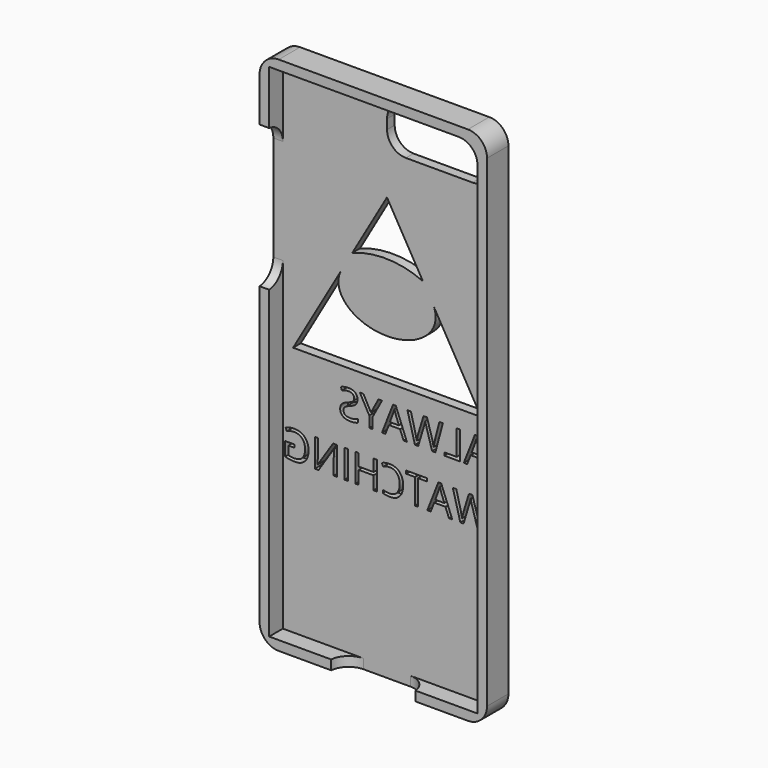
from build123d import *

# Parameters (mm, degrees)
F0_W          = 60.4104281297
F0_H          = 138.3
F1_DEPTH      = 3.55
F2_T          = -2.54
F3_R          = 5.08
F4_W          = 22.3621586338
F4_H          = 4.56
F5_DEPTH      = 25
F6_W          = 27.6652140649
F6_H          = 12.5321288562
F7_DEPTH      = 25
F8_R          = 5
F10_W         = 4.56
F10_H         = 37.7994477749
F11_DEPTH     = 25
F12_T1_DEPTH  = 2.54
F12_T3_DEPTH  = 2.54
F14_DEPTH     = 12.5
F15_TEXT_SIZE = 10.4652859995
F16_DEPTH     = 25


# Not quite as in the source:
# - a fillet or chamfer that OpenCascade refuses, or shapes differently, is made with other operations: its cross-section is extruded or revolved along the edge and cut away or added
# - Text() gives the source's letters only with a copy of the font that has no kerning and outlines rounded to 1/6400 em; it was checked with that copy


with BuildPart() as f1:
    # F0 (on Front) → F1 (new body, symmetric)
    with BuildSketch(Plane.XZ):
        Rectangle(F0_W, F0_H)
    extrude(amount=F1_DEPTH, both=True)

    # F2
    f2_openings = [f1.faces().sort_by_distance(p)[0] for p in [
        (0, -3.55, 0),
    ]]
    offset(amount=F2_T, openings=f2_openings)

    # F3
    f3_edges = [f1.edges().sort_by_distance(p)[0] for p in [
        (-30.205214, 0, 69.15),
        (30.205214, 0, 69.15),
        (-30.205214, 0, -69.15),
        (30.205214, 0, -69.15),
    ]]
    fillet(f3_edges, radius=F3_R)

    # F4 (on face) → F5 (cut)
    with BuildSketch(Plane.XY.offset(-66.61)):
        with Locations((-0.0060745515, -1.27)):
            Rectangle(F4_W, F4_H)
    extrude(amount=-F5_DEPTH, mode=Mode.SUBTRACT)

    # F6 (on face) → F7 (cut)
    with BuildSketch(Plane.XZ.offset(-1.01)):
        with Locations((13.8326070324, 60.3439355719)):
            Rectangle(F6_W, F6_H)
    extrude(amount=-F7_DEPTH, mode=Mode.SUBTRACT)

    # F8
    f8_edges = [f1.edges().sort_by_distance(p)[0] for p in [
        (0, 2.28, 54.077871),
        (0, 2.28, 66.61),
        (27.665214, 2.28, 54.077871),
        (27.665214, 0, 66.61),
    ]]
    fillet(f8_edges, radius=F8_R)

    # F10 (on face) → F11 (cut)
    with BuildSketch(Plane.YZ.offset(-27.6652140649)):
        with Locations((-1.27, 33.3837717772)):
            Rectangle(F10_W, F10_H)
    extrude(amount=-F11_DEPTH, mode=Mode.SUBTRACT)

    # F12: fillet of radius 5 on 4 edges, made by hand

    # F12_s2 → F12_t1 (join)
    with BuildSketch(Plane.YZ.offset(-30.2052140649)):
        with BuildLine():
            ThreePointArc((1.01, 47.3028932914), (-0.3021822171, 50.6792818946), (-3.55, 52.2834956646))
            Line((-3.55, 52.2834956646), (1.01, 52.2834956646))
            Line((1.01, 52.2834956646), (1.01, 47.3028932914))
        make_face()
        with BuildLine():
            ThreePointArc((-3.55, 14.4840478897), (-0.3021822171, 16.0882616597), (1.01, 19.4646502629))
            Line((1.01, 19.4646502629), (1.01, 14.4840478897))
            Line((1.01, 14.4840478897), (-3.55, 14.4840478897))
        make_face()
    extrude(amount=F12_T1_DEPTH)

    # F12_s4 → F12_t3 (join)
    with BuildSketch(Plane.XY.offset(-69.15)):
        with BuildLine():
            ThreePointArc((-11.1871538684, -3.55), (-9.5829400984, -0.3021822171), (-6.2065514952, 1.01))
            Line((-6.2065514952, 1.01), (-11.1871538684, 1.01))
            Line((-11.1871538684, 1.01), (-11.1871538684, -3.55))
        make_face()
        with BuildLine():
            ThreePointArc((6.1944023922, 1.01), (9.5707909954, -0.3021822171), (11.1750047654, -3.55))
            Line((11.1750047654, -3.55), (11.1750047654, 1.01))
            Line((11.1750047654, 1.01), (6.1944023922, 1.01))
        make_face()
    extrude(amount=F12_T3_DEPTH)

    # F13 (on face) → F14 (cut, symmetric)
    with BuildSketch(Plane(origin=(0, 3.55, 0), x_dir=(-1, 0, 0), z_dir=(0, 1, 0))):
        with BuildLine():
            Line((-12.4006852981, 21.7474929888), (-24.9808169901, 0))
            Line((-24.9808169901, 0), (24.9567557506, -0.0416752894))
            Line((24.9567557506, -0.0416752894), (12.3996804871, 21.7497956567))
            add(Edge.make_bspline(
                [(-12.4006852981, 21.7474929888), (-17.1778088292, 10.7942989213), (0.0018058911, 10.7958940167), (17.1814206113, 10.797489112), (12.3996804871, 21.7497956567)],
                knots=[6.0014017529, 6.0014017529, 6.0014017529, 7.8541215189, 7.8541215189, 9.7068412848, 9.7068412848, 9.7068412848], degree=2, weights=[1, 0.6007480055, 1, 0.6007480055, 1]))
        make_face()
        with BuildLine():
            Line((0.0240612395, 43.2263689521), (-9.5167658927, 26.7329747456))
            ThreePointArc((-9.5167658927, 26.7329747456), (-0.2052781768, 28.8342898459), (9.2129738133, 27.2799867593))
            Line((9.2129738133, 27.2799867593), (0.0240612395, 43.2263689521))
        make_face()
    extrude(amount=F14_DEPTH, both=True, mode=Mode.SUBTRACT)

    # F15 (on face) → F16 (cut)
    with BuildSketch(Plane(origin=(0, 3.55, 0), x_dir=(-1, 0, 0), z_dir=(0, 1, 0))):
        with Locations((-27.0157530904, -12.2214127332)):
            Text('ALWAYS', F15_TEXT_SIZE, font='Open Sans', text_align=(TextAlign.LEFT, TextAlign.BOTTOM))
        with Locations((-27.0157530904, -26.4542016925)):
            Text('WATCHING', F15_TEXT_SIZE, font='Open Sans', text_align=(TextAlign.LEFT, TextAlign.BOTTOM))
    extrude(amount=-F16_DEPTH, mode=Mode.SUBTRACT)


solid = f1.part
